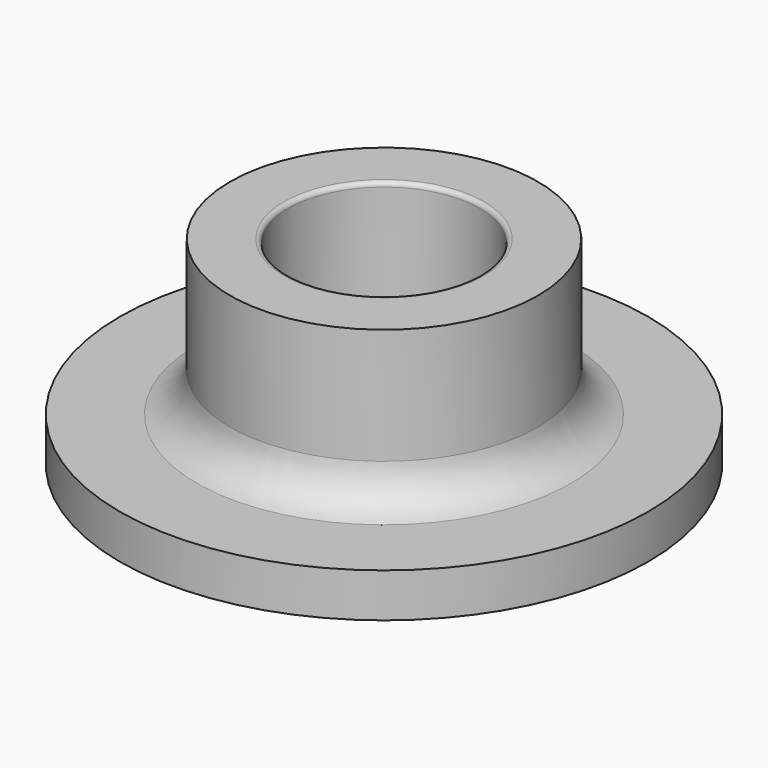
from build123d import *

# Parameters (mm, degrees)
F0_R     = 12
F0_R_2   = 7
F1_DEPTH = 2
F0_R_3   = 4.35
F2_DEPTH = 7.021
F8_R     = 0.2


with BuildPart() as f1:
    # F0 (on Top) → F1 (new body)
    with BuildSketch(Plane.XY):
        Circle(F0_R)
        Circle(F0_R_2, mode=Mode.SUBTRACT)
    extrude(amount=-F1_DEPTH)

    # F0 (on Top) → F2 (join)
    with BuildSketch(Plane.XY):
        Circle(F0_R_2)
        Circle(F0_R_3, mode=Mode.SUBTRACT)
    extrude(amount=F2_DEPTH)

    # F6 (on Front) → F7 (revolve)
    with BuildSketch(Plane.XZ):
        with BuildLine():
            ThreePointArc((-7, 1.7562480825), (-7.4708650568, 0.639716712), (-8.5, 0))
            Line((-8.5, 0), (-7, 0))
            Line((-7, 0), (-7, 1.7562480825))
        make_face()
    revolve(axis=Axis((0, 0, 5.6352536849), (0, 0, 1)))

    # F8
    f8_edges = [f1.edges().sort_by_distance(p)[0] for p in [
        (-4.35, 0, 7.021),
    ]]
    fillet(f8_edges, radius=F8_R)


solid = f1.part
